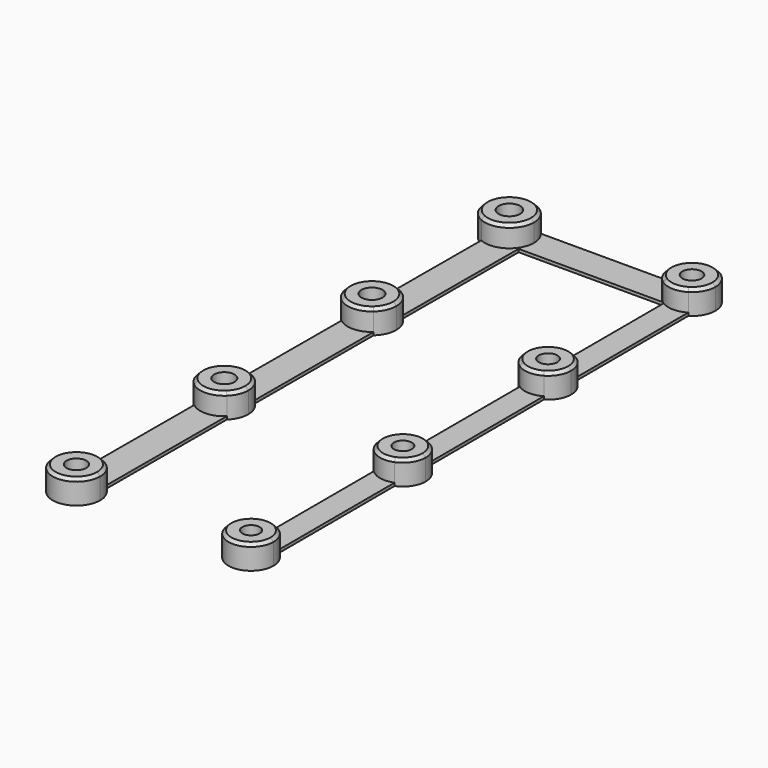
from build123d import *

# Parameters (mm, degrees)
F1_DEPTH = 0.5
F0_R     = 1.8
F0_R_2   = 1.75
F0_R_3   = 1.7
F0_R_4   = 1.65
F0_R_5   = 1.45
F0_R_6   = 1.5
F0_R_7   = 1.55
F0_R_8   = 1.6
F2_DEPTH = 4
F3_SIZE  = 0.5


# Not quite as in the source:
# - a feature names something its author has since deleted; it is built from what else it names


with BuildPart() as f1:
    # F0 (on Top) → F1 (new body)
    with BuildSketch(Plane.XY):
        with BuildLine():
            ThreePointArc((-34.4459491638, 25.172913447), (-33.7578745255, 23.955043307), (-33.5192581371, 22.5767412339))
            ThreePointArc((-33.5192581371, 22.5767412339), (-35.3994402039, 19.129654298), (-39.3155548901, 18.8441044547))
            Line((-39.3155548901, 18.8441044547), (-39.3856102198, -3.8797168626))
            ThreePointArc((-39.3856102198, -3.8797168626), (-36.7220470885, -2.9687824702), (-34.1081989909, -4.0138509584))
            Line((-34.1081989909, -4.0138509584), (-34.0341191547, 20.0153980404))
            Line((-34.0341191547, 20.0153980404), (-9.9966601452, 20.0153980404))
            ThreePointArc((-9.9966601452, 20.0153980404), (-11.4744909058, 22.4082296795), (-10.9585929746, 25.172913447))
            Line((-10.9585929746, 25.172913447), (-34.4459491638, 25.172913447))
        make_face()
    extrude(amount=F1_DEPTH)



with BuildPart() as f1b:
    # F0 (on Top) → F1, piece 2 (new body)
    with BuildSketch(Plane.XY):
        with BuildLine():
            ThreePointArc((-34.1267702169, -10.0377926374), (-36.747012257, -11.0667249351), (-39.4049081675, -10.1393850024))
            Line((-39.4049081675, -10.1393850024), (-39.4799453288, -34.4791611719))
            ThreePointArc((-39.4799453288, -34.4791611719), (-36.7996355415, -33.5950156167), (-34.2028031384, -34.7005631683))
            Line((-34.2028031384, -34.7005631683), (-34.1267702169, -10.0377926374))
        make_face()
    extrude(amount=F1_DEPTH)


with BuildPart() as f1c:
    # F0 (on Top) → F1, piece 3 (new body)
    with BuildSketch(Plane.XY):
        with BuildLine():
            Line((-5.5554180266, -3.69580099), (-5.5964215167, 19.8019486813))
            ThreePointArc((-5.5964215167, 19.8019486813), (-7.6604313925, 19.2233417208), (-9.7184515138, 19.8229048634))
            Line((-9.7184515138, 19.8229048634), (-9.6771501637, -3.8455385501))
            ThreePointArc((-9.6771501637, -3.8455385501), (-7.638026651, -3.1721760384), (-5.5554180266, -3.69580099))
        make_face()
    extrude(amount=F1_DEPTH)


with BuildPart() as f1d:
    # F0 (on Top) → F1, piece 4 (new body)
    with BuildSketch(Plane.XY):
        with BuildLine():
            ThreePointArc((-34.2206804706, -40.4994267733), (-36.8242800383, -41.5889418992), (-39.4990874596, -40.6882870387))
            Line((-39.4990874596, -40.6882870387), (-39.5762478682, -65.7167801383))
            ThreePointArc((-39.5762478682, -65.7167801383), (-36.9756537231, -64.6039381296), (-34.2978020361, -65.515320369))
            Line((-34.2978020361, -65.515320369), (-34.2206804706, -40.4994267733))
        make_face()
    extrude(amount=F1_DEPTH)


with BuildPart() as f1e:
    # F0 (on Top) → F1, piece 5 (new body)
    with BuildSketch(Plane.XY):
        with BuildLine():
            ThreePointArc((-5.5438297262, -10.3366742508), (-7.6245982257, -10.8675642808), (-9.6660593434, -10.2013223749))
            Line((-9.6660593434, -10.2013223749), (-9.6222940519, -35.2817694502))
            ThreePointArc((-9.6222940519, -35.2817694502), (-7.6890371511, -34.2390892716), (-5.5017688296, -34.440388773))
            Line((-5.5017688296, -34.440388773), (-5.5438297262, -10.3366742508))
        make_face()
    extrude(amount=F1_DEPTH)


with BuildPart() as f1f:
    # F0 (on Top) → F1, piece 6 (new body)
    with BuildSketch(Plane.XY):
        with BuildLine():
            ThreePointArc((-5.4894862388, -41.4791369772), (-7.6760387081, -41.6880687805), (-9.6129227708, -40.6521419841))
            Line((-9.6129227708, -40.6521419841), (-9.5691439378, -65.7403492338))
            ThreePointArc((-9.5691439378, -65.7403492338), (-7.5101002942, -65.1167253071), (-5.4471731405, -65.7273799451))
            Line((-5.4471731405, -65.7273799451), (-5.4894862388, -41.4791369772))
        make_face()
    extrude(amount=F1_DEPTH)


with BuildPart() as f1_1:
    add(f1.part)

    add(f1b.part)  # F2 merges F1b

    add(f1c.part)  # F2 merges F1c

    add(f1d.part)  # F2 merges F1d

    add(f1e.part)  # F2 merges F1e

    add(f1f.part)  # F2 merges F1f
    # F0 (on Top) → F2 (join)
    with BuildSketch(Plane.XY):
        with BuildLine():
            ThreePointArc((-39.3155548901, 18.8441044547), (-35.3994402039, 19.129654298), (-33.5192581371, 22.5767412339))
            ThreePointArc((-33.5192581371, 22.5767412339), (-33.7578745255, 23.955043307), (-34.4459491638, 25.172913447))
            ThreePointArc((-34.4459491638, 25.172913447), (-40.8686961023, 25.0769718053), (-39.3155548901, 18.8441044547))
        make_face()
        with Locations((-37.6192581371, 22.5767412339)):
            Circle(F0_R, mode=Mode.SUBTRACT)
        with BuildLine():
            ThreePointArc((-34.1081989909, -4.0138509584), (-36.7220470885, -2.9687824702), (-39.3856102198, -3.8797168626))
            ThreePointArc((-39.3856102198, -3.8797168626), (-40.8749320279, -7.0049892451), (-39.4049081675, -10.1393850024))
            ThreePointArc((-39.4049081675, -10.1393850024), (-36.747012257, -11.0667249351), (-34.1267702169, -10.0377926374))
            ThreePointArc((-34.1267702169, -10.0377926374), (-33.1283221824, -8.6719940136), (-32.774951274, -7.0174749417))
            ThreePointArc((-32.774951274, -7.0174749417), (-33.1232390521, -5.3743600258), (-34.1081989909, -4.0138509584))
        make_face()
        with Locations((-36.824951274, -7.0174749417)):
            Circle(F0_R_2, mode=Mode.SUBTRACT)
        with BuildLine():
            ThreePointArc((-34.2028031384, -34.7005631683), (-36.7996355415, -33.5950156167), (-39.4799453288, -34.4791611719))
            ThreePointArc((-39.4799453288, -34.4791611719), (-40.9672886463, -37.5791682773), (-39.4990874596, -40.6882870387))
            ThreePointArc((-39.4990874596, -40.6882870387), (-36.8242800383, -41.5889418992), (-34.2206804706, -40.4994267733))
            ThreePointArc((-34.2206804706, -40.4994267733), (-33.2939911195, -39.1747703785), (-32.9673076548, -37.5914998294))
            ThreePointArc((-32.9673076548, -37.5914998294), (-33.2891275297, -36.0195612278), (-34.2028031384, -34.7005631683))
        make_face()
        with Locations((-36.9673076548, -37.5914998294)):
            Circle(F0_R_3, mode=Mode.SUBTRACT)
        with BuildLine():
            ThreePointArc((-34.2978020361, -65.515320369), (-36.9756537231, -64.6039381296), (-39.5762478682, -65.7167801383))
            ThreePointArc((-39.5762478682, -65.7167801383), (-38.363689229, -72.18905184), (-32.8750057563, -68.5510643234))
            ThreePointArc((-32.8750057563, -68.5510643234), (-33.2483484695, -66.8747521053), (-34.2978020361, -65.515320369))
        make_face()
        with Locations((-36.8250057563, -68.5510643234)):
            Circle(F0_R_4, mode=Mode.SUBTRACT)
        with BuildLine():
            ThreePointArc((-5.4471731405, -65.7273799451), (-7.5101002942, -65.1167253071), (-9.5691439378, -65.7403492338))
            ThreePointArc((-9.5691439378, -65.7403492338), (-9.2726802717, -72.1703531716), (-3.7483014256, -68.8667067453))
            ThreePointArc((-3.7483014256, -68.8667067453), (-4.2002541951, -67.0819422046), (-5.4471731405, -65.7273799451))
        make_face()
        with Locations((-7.4983014256, -68.8667067453)):
            Circle(F0_R_5, mode=Mode.SUBTRACT)
        with BuildLine():
            ThreePointArc((-5.5017688296, -34.440388773), (-7.6890371511, -34.2390892716), (-9.6222940519, -35.2817694502))
            ThreePointArc((-9.6222940519, -35.2817694502), (-10.7287867634, -37.9688947195), (-9.6129227708, -40.6521419841))
            ThreePointArc((-9.6129227708, -40.6521419841), (-7.6760387081, -41.6880687805), (-5.4894862388, -41.4791369772))
            ThreePointArc((-5.4894862388, -41.4791369772), (-3.7736884319, -40.0801206812), (-3.1287925489, -37.962263743))
            ThreePointArc((-3.1287925489, -37.962263743), (-3.7773888828, -35.8389043921), (-5.5017688296, -34.440388773))
        make_face()
        with Locations((-6.9287925489, -37.962263743)):
            Circle(F0_R_6, mode=Mode.SUBTRACT)
        with BuildLine():
            ThreePointArc((-3.6482529968, -7.0196379713), (-4.1589106487, -5.1035762076), (-5.5554180266, -3.69580099))
            ThreePointArc((-5.5554180266, -3.69580099), (-7.638026651, -3.1721760384), (-9.6771501637, -3.8455385501))
            ThreePointArc((-9.6771501637, -3.8455385501), (-11.3482471352, -7.0263561975), (-9.6660593434, -10.2013223749))
            ThreePointArc((-9.6660593434, -10.2013223749), (-7.6245982257, -10.8675642808), (-5.5438297262, -10.3366742508))
            ThreePointArc((-5.5438297262, -10.3366742508), (-4.155572217, -8.9298696861), (-3.6482529968, -7.0196379713))
        make_face()
        with Locations((-7.4982529968, -7.0196379713)):
            Circle(F0_R_7, mode=Mode.SUBTRACT)
        with BuildLine():
            ThreePointArc((-3.7406042554, 23.1232913211), (-6.5752770767, 26.8749680133), (-10.9585929746, 25.172913447))
            ThreePointArc((-10.9585929746, 25.172913447), (-11.4744909058, 22.4082296795), (-9.9966601452, 20.0153980404))
            ThreePointArc((-9.9966601452, 20.0153980404), (-9.8596440675, 19.9161333406), (-9.7184515138, 19.8229048634))
            ThreePointArc((-9.7184515138, 19.8229048634), (-7.6604313925, 19.2233417208), (-5.5964215167, 19.8019486813))
            ThreePointArc((-5.5964215167, 19.8019486813), (-4.2360255237, 21.2209654658), (-3.7406042554, 23.1232913211))
        make_face()
        with Locations((-7.6406042554, 23.1232913211)):
            Circle(F0_R_8, mode=Mode.SUBTRACT)
    extrude(amount=F2_DEPTH)

    # F3
    f3_edges = [f1_1.edges().sort_by_distance(p)[0] for p in [
        (-41.719258, 22.576741, 4),
        (-34.244994, -3.895565, 4),
        (-34.45467, -40.703838, 4),
        (-34.073764, -71.385349, 4),
        (-11.540604, 23.123291, 4),
        (-9.441088, -10.343475, 4),
        (-8.355816, -41.484139, 4),
        (-9.54943, -72.006034, 4),
    ]]
    chamfer(f3_edges, length=F3_SIZE)


solid = f1_1.part
